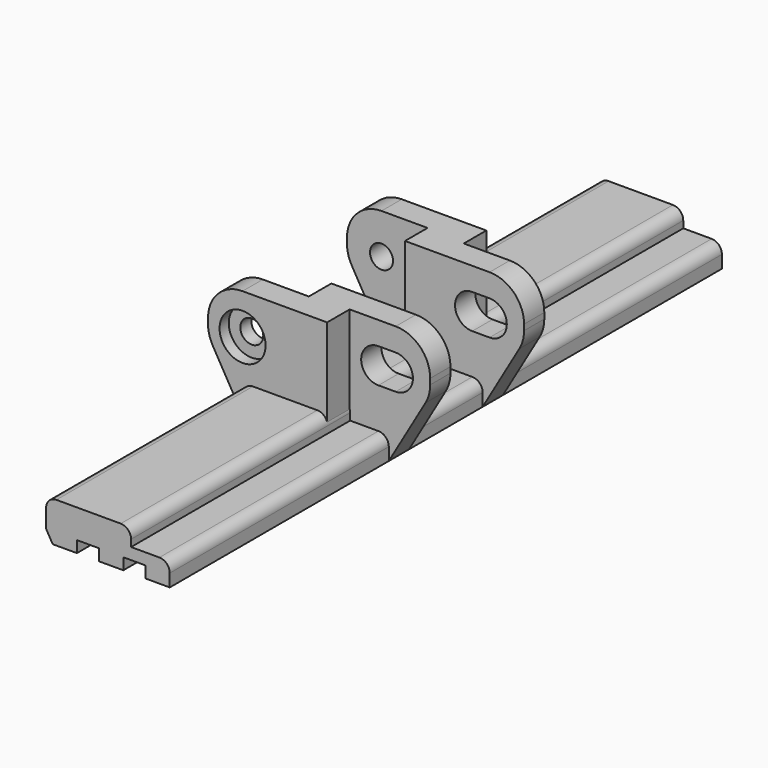
from build123d import *

# Parameters (mm, degrees)
F1_R      = 1
F2_DEPTH  = 2.2
F4_DEPTH  = 0.25
F6_DEPTH  = 2.2
F9_DEPTH  = 30
F11_DEPTH = 6.4
F13_R     = 2
F13_R_2   = 1
F14_DEPTH = 1


# Not quite as in the source:
# - a feature names something its author has since deleted; it is built from what else it names


with BuildPart() as f2:
    # F1 (on Front) → F2 (new body)
    with BuildSketch(Plane.XZ):
        with BuildLine():
            Line((7.35, 2), (7.35, 8.5))
            Line((7.35, 8.5), (0, 8.5))
            ThreePointArc((0, 8.5), (-2.1213203436, 7.6213203436), (-3, 5.5))
            Line((-3, 5.5), (-3, 5))
            ThreePointArc((-3, 5), (-2.8977774789, 4.2235428647), (-2.5980762114, 3.5))
            Line((-2.5980762114, 3.5), (-0.5775284417, 0.0003086038))
            Line((-0.5775284417, 0.0003086038), (0, -1))
            Line((0, -1), (0, 0))
            Line((0, 0), (2, 0))
            Line((2, 0), (7.35, 0))
            Line((7.35, 0), (7.35, 2))
        make_face()
        with Locations((0, 5)):
            Circle(F1_R, mode=Mode.SUBTRACT)
    extrude(amount=-F2_DEPTH)

    # F3 (on Front) → F4 (join)
    with BuildSketch(Plane.XZ):
        Polygon((7.35, 8.5), (4, 8.5), (4, 2), (4, 0), (7.35, 0), (7.35, 2), align=None)
    extrude(amount=F4_DEPTH)

    # F5 (on face) → F6 (join)
    with BuildSketch(Plane.XZ.offset(0.25)):
        with BuildLine():
            ThreePointArc((13.9434358481, 3.491991213), (14.2465762155, 4.2190734812), (14.35, 5))
            Line((14.35, 5), (14.35, 5.5))
            ThreePointArc((14.35, 5.5), (13.4713203436, 7.6213203436), (11.35, 8.5))
            Line((11.35, 8.5), (4, 8.5))
            Line((4, 8.5), (4, 2))
            Line((4, 2), (4, 0))
            Line((4, 0), (7.3888939805, 0))
            Line((7.3888939805, 0), (10.75, -1))
            Line((10.75, -1), (10.75, -2))
            Line((10.75, -2), (13.9434358481, 3.491991213))
        make_face()
        with BuildLine():
            Line((11.35, 3.5), (9.85, 3.5))
            ThreePointArc((9.85, 3.5), (8.35, 5), (9.85, 6.5))
            Line((9.85, 6.5), (11.35, 6.5))
            ThreePointArc((11.35, 6.5), (12.85, 5), (11.35, 3.5))
        make_face(mode=Mode.SUBTRACT)
    extrude(amount=F6_DEPTH)

    # F8 (on offset) → F9 (join)
    with BuildSketch(Plane.XZ.offset(6.45)):
        with BuildLine():
            Line((10.75, -2), (10.75, -1))
            Line((10.75, -1), (10.75, -0.9))
            ThreePointArc((10.75, -0.9), (10.4863961031, -0.2636038969), (9.85, 0))
            Line((9.85, 0), (7.3888939805, 0))
            Line((7.3888939805, 0), (7.3888939805, 0.6))
            ThreePointArc((7.3888939805, 0.6), (7.1252900836, 1.2363961031), (6.4888939805, 1.5))
            Line((6.4888939805, 1.5), (0.9, 1.5))
            ThreePointArc((0.9, 1.5), (0.2636038969, 1.2363961031), (0, 0.6))
            Line((0, 0.6), (0, -1))
            Line((0, -1), (0.5773502692, -2))
            Line((0.5773502692, -2), (2.6773502692, -2))
            Line((2.6773502692, -2), (2.6773502692, -1))
            Line((2.6773502692, -1), (4.6136751346, -1))
            Line((4.6136751346, -1), (4.6136751346, -2))
            Line((4.6136751346, -2), (6.7136751346, -2))
            Line((6.7136751346, -2), (6.7136751346, -1))
            Line((6.7136751346, -1), (8.65, -1))
            Line((8.65, -1), (8.65, -2))
            Line((8.65, -2), (10.75, -2))
        make_face()
    extrude(amount=-F9_DEPTH)

    # F10 (on offset) → F11 (cut)
    with BuildSketch(Plane.XZ.offset(6.45)):
        with BuildLine():
            ThreePointArc((0.9, 1.5), (0.2636038969, 1.2363961031), (0, 0.6))
            Line((0, 0.6), (0, -1))
            Line((0, -1), (0.5773502692, -2))
            Line((0.5773502692, -2), (2.0773502692, -2))
            Line((2.0773502692, -2), (2.0773502692, -0.8))
            Line((2.0773502692, -0.8), (3.6773515204, 1.5))
            Line((3.6773515204, 1.5), (0.9, 1.5))
        make_face()
    extrude(amount=-F11_DEPTH, mode=Mode.SUBTRACT)

    # F12: F2 across plane


with BuildPart() as f2_1:
    add(f2.part)
    add(f2.part.mirror(Plane(origin=(8.5554041441, -6.45, 4.0498921838), x_dir=(1, 0, 0), z_dir=(0, -1, 0))))

    # F13 (on face) → F14 (cut)
    with BuildSketch(Plane.XZ.offset(15.1)):
        with Locations((0, 5)):
            Circle(F13_R)
        with Locations((0, 5)):
            Circle(F13_R_2, mode=Mode.SUBTRACT)
    extrude(amount=-F14_DEPTH, mode=Mode.SUBTRACT)


solid = f2_1.part
